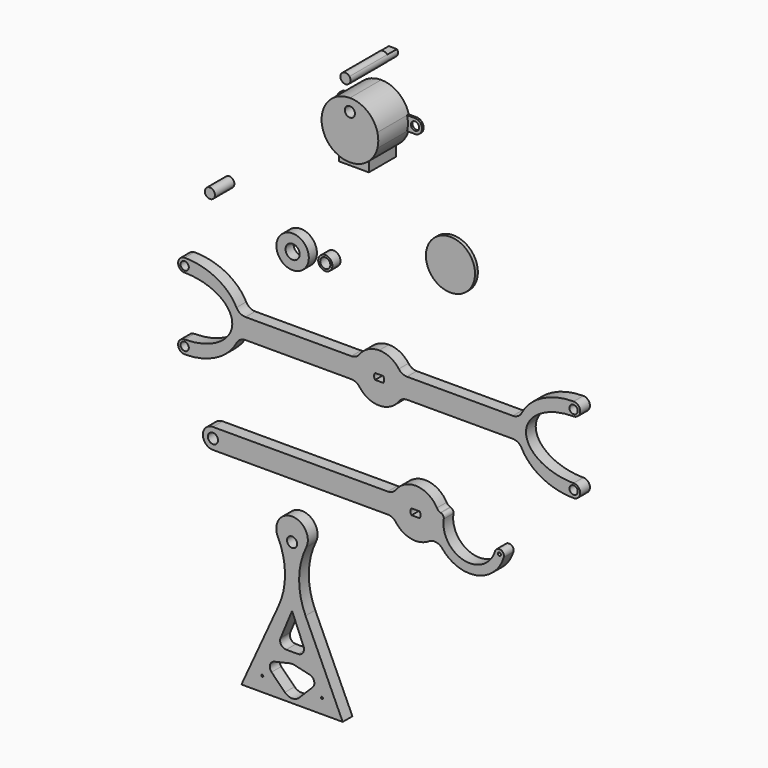
from build123d import *

# Parameters (mm, degrees)
F0_R      = 12.13
F1_DEPTH  = 1.75
F2_R      = 2.05
F3_DEPTH  = 6
F4_R      = 2.5
F5_DEPTH  = 12
F6_R      = 8
F6_R_2    = 3.5
F7_DEPTH  = 5
F8_R      = 3.5
F8_R_2    = 2.5
F9_DEPTH  = 5
F10_R     = 0.5
F10_R_2   = 2.5
F11_DEPTH = 6
F12_R     = 2.05
F13_DEPTH = 1
F12_R_2   = 2.5
F14_DEPTH = 19.3
F15_DEPTH = 16.8
F16_DEPTH = 1.7
F18_DEPTH = 23.3
F19_DEPTH = 29.3
F20_R     = 0.75
F20_R_2   = 2.5
F21_DEPTH = 6


# Not quite as in the source:
# - a feature names something its author has since deleted; it is built from what else it names


with BuildPart() as f1:
    # F0 (on Front) → F1 (new body)
    with BuildSketch(Plane.XZ):
        with Locations((49.7920177877, 38.1558388472)):
            Circle(F0_R)
    extrude(amount=F1_DEPTH)


with BuildPart() as f3:
    # F2 (on Front) → F3 (new body)
    with BuildSketch(Plane.XZ):
        with BuildLine():
            Line((4.2344670436, -14.6548693209), (-47.9935154794, -14.6548693209))
            ThreePointArc((-47.9935154794, -14.6548693209), (-50.5941906078, -13.9252895434), (-52.4359057436, -11.9494648715))
            add(Edge.make_bspline(
                [(-52.4359057436, -11.9494648715), (-59.3028665424, 1.3451306791), (-78.0178058715, 1.3451306791)],
                knots=[0.3757002438, 0.3757002438, 0.3757002438, 1.5707963268, 1.5707963268, 1.5707963268], degree=2, weights=[1, 0.8267176124, 1]))
            ThreePointArc((-78.0178058715, 1.3451306791), (-81.2678058715, -1.9048693209), (-78.0178058715, -5.1548693209))
            add(Edge.make_bspline(
                [(-78.0178058715, -34.1548693209), (-54.5178058715, -34.1548693209), (-54.5178058715, -19.6548693209), (-54.5178058715, -5.1548693209), (-78.0178058715, -5.1548693209)],
                knots=[1.5707963268, 1.5707963268, 1.5707963268, 3.1415926536, 3.1415926536, 4.7123889804, 4.7123889804, 4.7123889804], degree=2, weights=[1, 0.7071067812, 1, 0.7071067812, 1]))
            ThreePointArc((-78.0178058715, -34.1548693209), (-81.2678058715, -37.4048693209), (-78.0178058715, -40.6548693209))
            add(Edge.make_bspline(
                [(-78.0178058715, -40.6548693209), (-59.3028665424, -40.6548693209), (-52.4359057436, -27.3602737703)],
                knots=[4.7123889804, 4.7123889804, 4.7123889804, 5.9074850634, 5.9074850634, 5.9074850634], degree=2, weights=[1, 0.8267176124, 1]))
            ThreePointArc((-52.4359057436, -27.3602737703), (-50.5941906078, -25.3844490985), (-47.9935154794, -24.6548693209))
            Line((-47.9935154794, -24.6548693209), (4.2344670436, -24.6548693209))
            ThreePointArc((4.2344670436, -24.6548693209), (6.5031800761, -25.1992053775), (8.2779161863, -26.7136928503))
            ThreePointArc((8.2779161863, -26.7136928503), (12.5372828507, -30.3484627851), (17.9821941285, -31.6548693209))
            Line((17.9821941285, -31.6548693209), (17.9821941285, -21.1548693209))
            Line((17.9821941285, -21.1548693209), (15.9821941285, -21.1548693209))
            ThreePointArc((15.9821941285, -21.1548693209), (15.4821941285, -19.6548693209), (15.9821941285, -18.1548693209))
            Line((15.9821941285, -18.1548693209), (17.9821941285, -18.1548693209))
            Line((17.9821941285, -18.1548693209), (17.9821941285, -7.6548693209))
            ThreePointArc((17.9821941285, -7.6548693209), (12.5372828507, -8.9612758568), (8.2779161863, -12.5960457915))
            ThreePointArc((8.2779161863, -12.5960457915), (6.5031800761, -14.1105332643), (4.2344670436, -14.6548693209))
        make_face()
        with Locations((-78.0178058715, -37.1548693209)):
            Circle(F2_R, mode=Mode.SUBTRACT)
        with Locations((-78.0178058715, -2.1548693209)):
            Circle(F2_R, mode=Mode.SUBTRACT)
        with BuildLine():
            ThreePointArc((27.6864720708, -12.5960457915), (23.4271054064, -8.9612758568), (17.9821941285, -7.6548693209))
            Line((17.9821941285, -7.6548693209), (17.9821941285, -18.1548693209))
            Line((17.9821941285, -18.1548693209), (19.9821941285, -18.1548693209))
            ThreePointArc((19.9821941285, -18.1548693209), (20.4821941285, -19.6548693209), (19.9821941285, -21.1548693209))
            Line((19.9821941285, -21.1548693209), (17.9821941285, -21.1548693209))
            Line((17.9821941285, -21.1548693209), (17.9821941285, -31.6548693209))
            ThreePointArc((17.9821941285, -31.6548693209), (23.4271054064, -30.3484627851), (27.6864720708, -26.7136928503))
            ThreePointArc((27.6864720708, -26.7136928503), (29.4612081809, -25.1992053775), (31.7299212134, -24.6548693209))
            Line((31.7299212134, -24.6548693209), (83.9579037364, -24.6548693209))
            ThreePointArc((83.9579037364, -24.6548693209), (86.5585788648, -25.3844490985), (88.4002940006, -27.3602737703))
            add(Edge.make_bspline(
                [(88.4002940006, -27.3602737703), (95.2672547995, -40.6548693209), (113.9821941285, -40.6548693209)],
                knots=[3.5172928974, 3.5172928974, 3.5172928974, 4.7123889804, 4.7123889804, 4.7123889804], degree=2, weights=[1, 0.8267176124, 1]))
            ThreePointArc((113.9821941285, -40.6548693209), (117.2321941285, -37.4048693209), (113.9821941285, -34.1548693209))
            add(Edge.make_bspline(
                [(113.9821941285, -5.1548693209), (90.4821941285, -5.1548693209), (90.4821941285, -19.6548693209), (90.4821941285, -34.1548693209), (113.9821941285, -34.1548693209)],
                knots=[1.5707963268, 1.5707963268, 1.5707963268, 3.1415926536, 3.1415926536, 4.7123889804, 4.7123889804, 4.7123889804], degree=2, weights=[1, 0.7071067812, 1, 0.7071067812, 1]))
            ThreePointArc((113.9821941285, -5.1548693209), (117.2321941285, -1.9048693209), (113.9821941285, 1.3451306791))
            add(Edge.make_bspline(
                [(113.9821941285, 1.3451306791), (95.2672547995, 1.3451306791), (88.4002940006, -11.9494648715)],
                knots=[1.5707963268, 1.5707963268, 1.5707963268, 2.7658924098, 2.7658924098, 2.7658924098], degree=2, weights=[1, 0.8267176124, 1]))
            ThreePointArc((88.4002940006, -11.9494648715), (86.5585788648, -13.9252895434), (83.9579037364, -14.6548693209))
            Line((83.9579037364, -14.6548693209), (31.7299212134, -14.6548693209))
            ThreePointArc((31.7299212134, -14.6548693209), (29.4612081809, -14.1105332643), (27.6864720708, -12.5960457915))
        make_face()
        with Locations((113.9821941285, -37.1548693209)):
            Circle(F2_R, mode=Mode.SUBTRACT)
        with Locations((113.9821941285, -2.1548693209)):
            Circle(F2_R, mode=Mode.SUBTRACT)
    extrude(amount=F3_DEPTH)


with BuildPart() as f5:
    # F4 (on Front) → F5 (new body)
    with BuildSketch(Plane.XZ):
        with Locations((-60.7640594244, 37.4355688691)):
            Circle(F4_R)
    extrude(amount=F5_DEPTH)


with BuildPart() as f7:
    # F6 (on Front) → F7 (new body)
    with BuildSketch(Plane.XZ):
        with Locations((-25.5331490189, 20.5946248025)):
            Circle(F6_R)
        with Locations((-25.5331490189, 20.5946248025)):
            Circle(F6_R_2, mode=Mode.SUBTRACT)
    extrude(amount=F7_DEPTH)


with BuildPart() as f9:
    # F8 (on Front) → F9 (new body)
    with BuildSketch(Plane.XZ):
        with Locations((-9.3970168382, 20.9394581616)):
            Circle(F8_R)
        with Locations((-9.3970168382, 20.9394581616)):
            Circle(F8_R_2, mode=Mode.SUBTRACT)
    extrude(amount=F9_DEPTH)


with BuildPart() as f11:
    # F10 (on Front) → F11 (new body)
    with BuildSketch(Plane.XZ):
        with BuildLine():
            Line((-31.6467687653, -134.8523066742), (-50, -175))
            Line((-50, -175), (0, -175))
            Line((0, -175), (-18.3532312347, -134.8523066742))
            ThreePointArc((-18.3532312347, -134.8523066742), (-21.5191746525, -119.88660208), (-18, -105))
            ThreePointArc((-18, -105), (-25, -93.814384451), (-32, -105))
            ThreePointArc((-32, -105), (-28.4808253475, -119.88660208), (-31.6467687653, -134.8523066742))
        make_face()
        with Locations((-39.7090827208, -167.9052151838)):
            Circle(F10_R, mode=Mode.SUBTRACT)
        with BuildLine():
            Line((-28.5473133889, -171.4289302292), (-35.1352190008, -164.7969053686))
            ThreePointArc((-35.1352190008, -164.7969053686), (-35.8888128999, -161.8495016053), (-33.6787390246, -159.7588877781))
            Line((-33.6787390246, -159.7588877781), (-26.1198467618, -158.0217988936))
            ThreePointArc((-26.1198467618, -158.0217988936), (-25, -157.8947798324), (-23.8801532382, -158.0217988936))
            Line((-23.8801532382, -158.0217988936), (-16.3212609754, -159.7588877781))
            ThreePointArc((-16.3212609754, -159.7588877781), (-14.1111871001, -161.8495016053), (-14.8647809992, -164.7969053686))
            Line((-14.8647809992, -164.7969053686), (-21.4526866111, -171.4289302292))
            ThreePointArc((-21.4526866111, -171.4289302292), (-25, -172.9052151838), (-28.5473133889, -171.4289302292))
        make_face(mode=Mode.SUBTRACT)
        with Locations((-10.2909172792, -167.9052151838)):
            Circle(F10_R, mode=Mode.SUBTRACT)
        with BuildLine():
            Line((-30.6722089534, -148.5158730066), (-25, -134.8523066742))
            Line((-25, -134.8523066742), (-19.3277910466, -148.5158730066))
            ThreePointArc((-19.3277910466, -148.5158730066), (-19.6034642215, -151.3318306011), (-22.0985272688, -152.6660994134))
            Line((-22.0985272688, -152.6660994134), (-27.9014727312, -152.6660994134))
            ThreePointArc((-27.9014727312, -152.6660994134), (-30.3965357785, -151.3318306011), (-30.6722089534, -148.5158730066))
        make_face(mode=Mode.SUBTRACT)
        with Locations((-25, -105)):
            Circle(F10_R_2, mode=Mode.SUBTRACT)
    extrude(amount=F11_DEPTH)


with BuildPart() as f13:
    # F12 (on Front) → F13 (new body)
    with BuildSketch(Plane.XZ):
        with BuildLine():
            Line((31.7033928931, 95.6584931427), (27.771646281, 95.6584931427))
            ThreePointArc((27.771646281, 95.6584931427), (28.2033928931, 92.2084931427), (27.771646281, 88.7584931427))
            Line((27.771646281, 88.7584931427), (31.7533929121, 88.7590366495))
            ThreePointArc((31.7533929121, 88.7590366495), (34.1603346184, 89.7867045654), (35.1533928693, 92.2081308049))
            Line((35.153392874, 92.2081308049), (35.1533928931, 92.2083119738))
            ThreePointArc((35.1533928883, 92.2083119738), (34.1429753402, 94.6479474841), (31.7033928931, 95.6584931427))
        make_face()
        with Locations((31.7033928931, 92.2084931427)):
            Circle(F12_R, mode=Mode.SUBTRACT)
    extrude(amount=F13_DEPTH)



with BuildPart() as f13b:
    # F12 (on Front) → F13, piece 2 (new body)
    with BuildSketch(Plane.XZ):
        with BuildLine():
            ThreePointArc((0.6351395051, 88.7584931427), (0.2033928931, 92.2084931427), (0.6351395051, 95.6584931427))
            Line((0.6351395051, 95.6584931427), (-3.2966071069, 95.6584931427))
            ThreePointArc((-3.2966071069, 95.6584931427), (-5.7361895541, 94.6479474841), (-6.7466071022, 92.2083119738))
            Line((-6.7466071069, 92.2083119738), (-6.7466070879, 92.2081308049))
            ThreePointArc((-6.7466070831, 92.2081308049), (-5.7535488323, 89.7867045654), (-3.346607126, 88.7590366495))
            Line((-3.346607126, 88.7590366495), (0.6351395051, 88.7584931427))
        make_face()
        with Locations((-3.2966071069, 92.2084931427)):
            Circle(F12_R, mode=Mode.SUBTRACT)
    extrude(amount=F13_DEPTH)


with BuildPart() as f13_1:
    add(f13.part)

    add(f13b.part)  # F14 merges F13b
    # F12 (on Front) → F14 (join)
    with BuildSketch(Plane.XZ):
        with BuildLine():
            ThreePointArc((27.771646281, 95.6584931427), (22.7969951645, 103.260642255), (14.2033928931, 106.2084931427))
            ThreePointArc((14.2033928931, 106.2084931427), (5.6097906216, 103.260642255), (0.6351395051, 95.6584931427))
            ThreePointArc((0.6351395051, 95.6584931427), (0.2033928931, 92.2084931427), (0.6351395051, 88.7584931427))
            ThreePointArc((0.6351395051, 88.7584931427), (2.9202544808, 83.9205025799), (6.8533928931, 80.2930619713))
            ThreePointArc((6.8533928931, 80.2930619713), (10.3834476316, 78.7397137548), (14.2033928931, 78.2084931427))
            ThreePointArc((14.2033928931, 78.2084931427), (18.0233381545, 78.7397137548), (21.5533928931, 80.2930619713))
            ThreePointArc((21.5533928931, 80.2930619713), (25.4865313053, 83.9205025799), (27.771646281, 88.7584931427))
            ThreePointArc((27.771646281, 88.7584931427), (28.2033928931, 92.2084931427), (27.771646281, 95.6584931427))
        make_face()
        with BuildLine():
            ThreePointArc((14.2033928931, 95.6084931427), (9.6033928931, 100.2084931427), (14.2033928931, 104.8084931427))
            ThreePointArc((14.2033928931, 104.8084931427), (18.8033928931, 100.2084931427), (14.2033928931, 95.6084931427))
        make_face(mode=Mode.SUBTRACT)
        with BuildLine():
            ThreePointArc((14.2033928931, 95.6084931427), (18.8033928931, 100.2084931427), (14.2033928931, 104.8084931427))
            ThreePointArc((14.2033928931, 104.8084931427), (9.6033928931, 100.2084931427), (14.2033928931, 95.6084931427))
        make_face()
        with Locations((14.1654592007, 100.134126842)):
            Circle(F12_R_2, mode=Mode.SUBTRACT)
    extrude(amount=F14_DEPTH)

    # F12 (on Front) → F15 (join)
    with BuildSketch(Plane.XZ):
        with BuildLine():
            ThreePointArc((14.2033928931, 78.2084931427), (10.3834476316, 78.7397137548), (6.8533928931, 80.2930619713))
            Line((6.8533928931, 80.2930619713), (6.8533928931, 75.2084931427))
            Line((6.8533928931, 75.2084931427), (14.2033928931, 75.2084931427))
            Line((14.2033928931, 75.2084931427), (21.5533928931, 75.2084931427))
            Line((21.5533928931, 75.2084931427), (21.5533928931, 80.2930619713))
            ThreePointArc((21.5533928931, 80.2930619713), (18.0233381545, 78.7397137548), (14.2033928931, 78.2084931427))
        make_face()
    extrude(amount=F15_DEPTH)

    # F12 (on Front) → F16 (join)
    with BuildSketch(Plane.XZ):
        with BuildLine():
            ThreePointArc((14.2033928931, 95.6084931427), (18.8033928931, 100.2084931427), (14.2033928931, 104.8084931427))
            ThreePointArc((14.2033928931, 104.8084931427), (9.6033928931, 100.2084931427), (14.2033928931, 95.6084931427))
        make_face()
        with Locations((14.1654592007, 100.134126842)):
            Circle(F12_R_2, mode=Mode.SUBTRACT)
    extrude(amount=-F16_DEPTH)


with BuildPart() as f18:
    # F17 (on Front) → F18 (new body)
    with BuildSketch(Plane.XZ):
        with BuildLine():
            Line((-3.4609997291, 99.5840311646), (-5.4609997291, 99.5840311646))
            ThreePointArc((-5.4609997291, 99.5840311646), (-4.5790337179, 98.8479631871), (-3.4609997291, 98.5840311646))
            ThreePointArc((-3.4609997291, 98.5840311646), (-2.3429657404, 98.8479631871), (-1.4609997291, 99.5840311646))
            Line((-1.4609997291, 99.5840311646), (-3.4609997291, 99.5840311646))
        make_face()
    extrude(amount=-F18_DEPTH)



with BuildPart() as f18b:
    # F17 (on Front) → F18, piece 2 (new body)
    with BuildSketch(Plane.XZ):
        with BuildLine():
            ThreePointArc((-1.4609997291, 102.5840311646), (-2.3429657404, 103.3200991421), (-3.4609997291, 103.5840311646))
            ThreePointArc((-3.4609997291, 103.5840311646), (-4.5790337179, 103.3200991421), (-5.4609997291, 102.5840311646))
            Line((-5.4609997291, 102.5840311646), (-3.4609997291, 102.5840311646))
            Line((-3.4609997291, 102.5840311646), (-1.4609997291, 102.5840311646))
        make_face()
    extrude(amount=-F18_DEPTH)


with BuildPart() as f18_1:
    add(f18.part)

    add(f18b.part)  # F19 merges F18b
    # F17 (on Front) → F19 (join)
    with BuildSketch(Plane.XZ):
        with BuildLine():
            Line((-3.4609997291, 102.5840311646), (-5.4609997291, 102.5840311646))
            ThreePointArc((-5.4609997291, 102.5840311646), (-5.9609997291, 101.0840311646), (-5.4609997291, 99.5840311646))
            Line((-5.4609997291, 99.5840311646), (-3.4609997291, 99.5840311646))
            Line((-3.4609997291, 99.5840311646), (-1.4609997291, 99.5840311646))
            ThreePointArc((-1.4609997291, 99.5840311646), (-0.9609997291, 101.0840311646), (-1.4609997291, 102.5840311646))
            Line((-1.4609997291, 102.5840311646), (-3.4609997291, 102.5840311646))
        make_face()
    extrude(amount=-F19_DEPTH)


with BuildPart() as f21:
    # F20 (on Front) → F21 (new body)
    with BuildSketch(Plane.XZ):
        with BuildLine():
            Line((22.2055752763, -67.634176104), (-64.0466976388, -67.634176104))
            ThreePointArc((-64.0466976388, -67.634176104), (-67.5822315448, -69.0986421981), (-69.0466976388, -72.634176104))
            ThreePointArc((-69.0466976388, -72.634176104), (-67.5822315448, -76.16971001), (-64.0466976388, -77.634176104))
            Line((-64.0466976388, -77.634176104), (22.2055752763, -77.634176104))
            ThreePointArc((22.2055752763, -77.634176104), (24.4742883087, -78.1785121606), (26.2490244189, -79.6929996335))
            ThreePointArc((26.2490244189, -79.6929996335), (33.7982610449, -84.4390817337), (42.5375035381, -82.666538481))
            ThreePointArc((42.5375035381, -82.666538481), (46.0436948987, -81.905214437), (49.1571188057, -83.6883531675))
            ThreePointArc((49.1571188057, -83.6883531675), (66.1486296958, -89.7957793237), (79.4943220237, -77.634176104))
            ThreePointArc((79.4943220237, -77.634176104), (77.9809707596, -74.8351105543), (75.1819052099, -76.3484618183))
            ThreePointArc((75.1819052099, -76.3484618183), (59.8502264198, -85.3126028522), (49.8817162799, -70.614133388))
            ThreePointArc((49.8817162799, -70.614133388), (49.5978451418, -69.2367315021), (48.4774377879, -68.3867278905))
            Line((48.4774377879, -68.3867278905), (48.2625933234, -68.3226736469))
            ThreePointArc((48.2625933234, -68.3226736469), (47.2322808004, -67.779576481), (46.4864494167, -66.8850185043))
            ThreePointArc((46.4864494167, -66.8850185043), (36.7282618527, -60.6592256747), (26.2490244189, -65.5753525746))
            ThreePointArc((26.2490244189, -65.5753525746), (24.4742883087, -67.0898400474), (22.2055752763, -67.634176104))
        make_face()
        with Locations((77.3381136168, -76.9913189612)):
            Circle(F20_R, mode=Mode.SUBTRACT)
        with Locations((-64.0466976388, -72.634176104)):
            Circle(F20_R_2, mode=Mode.SUBTRACT)
        with BuildLine():
            ThreePointArc((33.9533023612, -74.134176104), (33.4533023612, -72.634176104), (33.9533023612, -71.134176104))
            Line((33.9533023612, -71.134176104), (37.9533023612, -71.134176104))
            ThreePointArc((37.9533023612, -71.134176104), (38.4533023612, -72.634176104), (37.9533023612, -74.134176104))
            Line((37.9533023612, -74.134176104), (33.9533023612, -74.134176104))
        make_face(mode=Mode.SUBTRACT)
    extrude(amount=F21_DEPTH)


solid = Compound([f1.part, f3.part, f5.part, f7.part, f9.part, f11.part, f13_1.part, f18_1.part, f21.part])
